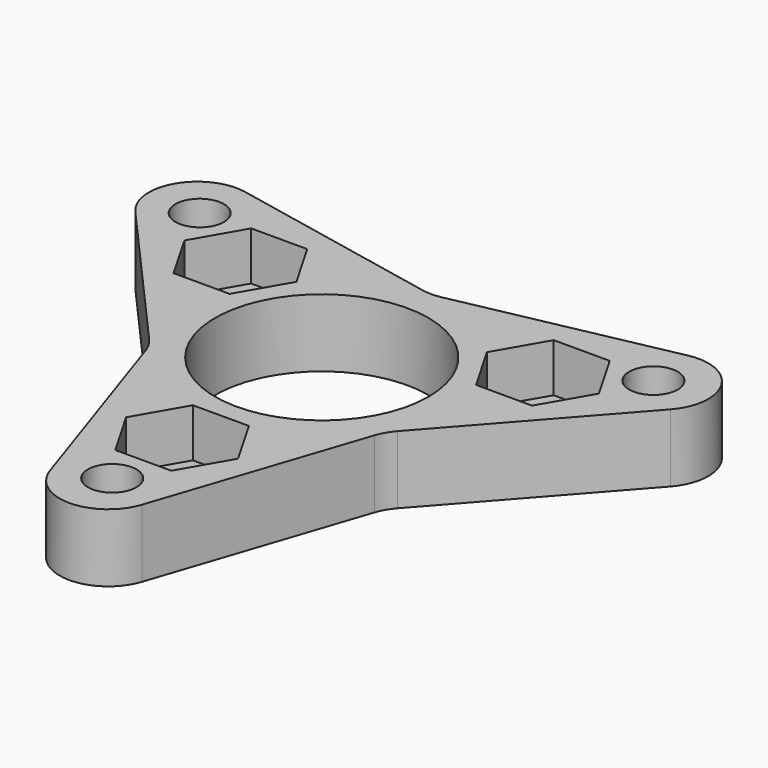
from build123d import *

# Parameters (mm, degrees)
F0_R     = 2.5
F0_R_2   = 11
F1_DEPTH = 7
F0_R_3   = 3.5
F2_DEPTH = 2
F3_R     = 5


# Not quite as in the source:
# - a feature names something its author has since deleted; it is built from what else it names


with BuildPart() as f1:
    # F0 (on Top) → F1 (new body)
    with BuildSketch(Plane.XY):
        Polygon((0, 14), (-37.5, 21.6506350946), (-12.124355653, -7), (0, -43.3012701892), (12.124355653, -7), (37.5, 21.6506350946), align=None)
        with Locations((0, -27)):
            Circle(F0_R, mode=Mode.SUBTRACT)
        Polygon((2.8867513459, -13), (5.7735026919, -18), (2.8867513459, -23), (-2.8867513459, -23), (-5.7735026919, -18), (-2.8867513459, -13), align=None, mode=Mode.SUBTRACT)
        with Locations((-23.3826859022, 13.5)):
            Circle(F0_R, mode=Mode.SUBTRACT)
        Polygon((-12.7017059222, 4), (-18.4752086141, 4), (-21.36195996, 9), (-18.4752086141, 14), (-12.7017059222, 14), (-9.8149545762, 9), align=None, mode=Mode.SUBTRACT)
        Circle(F0_R_2, mode=Mode.SUBTRACT)
        Polygon((21.36195996, 9), (18.4752086141, 4), (12.7017059222, 4), (9.8149545762, 9), (12.7017059222, 14), (18.4752086141, 14), align=None, mode=Mode.SUBTRACT)
        with Locations((23.3826859022, 13.5)):
            Circle(F0_R, mode=Mode.SUBTRACT)
    extrude(amount=F1_DEPTH)

    # F0 (on Top) → F2 (join)
    with BuildSketch(Plane.XY):
        Polygon((-21.36195996, 9), (-18.4752086141, 4), (-12.7017059222, 4), (-9.8149545762, 9), (-12.7017059222, 14), (-18.4752086141, 14), align=None)
        with Locations((-15.5884572681, 9)):
            Circle(F0_R_3, mode=Mode.SUBTRACT)
        Polygon((2.8867513459, -23), (5.7735026919, -18), (2.8867513459, -13), (-2.8867513459, -13), (-5.7735026919, -18), (-2.8867513459, -23), align=None)
        with Locations((0, -18)):
            Circle(F0_R_3, mode=Mode.SUBTRACT)
        Polygon((12.7017059222, 4), (18.4752086141, 4), (21.36195996, 9), (18.4752086141, 14), (12.7017059222, 14), (9.8149545762, 9), align=None)
        with Locations((15.5884572681, 9)):
            Circle(F0_R_3, mode=Mode.SUBTRACT)
    extrude(amount=F2_DEPTH)

    # F3
    f3_edges = [f1.edges().sort_by_distance(p)[0] for p in [
        (37.5, 21.650635, 3.5),
        (-37.5, 21.650635, 3.5),
        (0, -43.30127, 3.5),
        (-12.124356, -7, 3.5),
        (0, 14, 3.5),
        (12.124356, -7, 3.5),
    ]]
    fillet(f3_edges, radius=F3_R)


solid = f1.part
